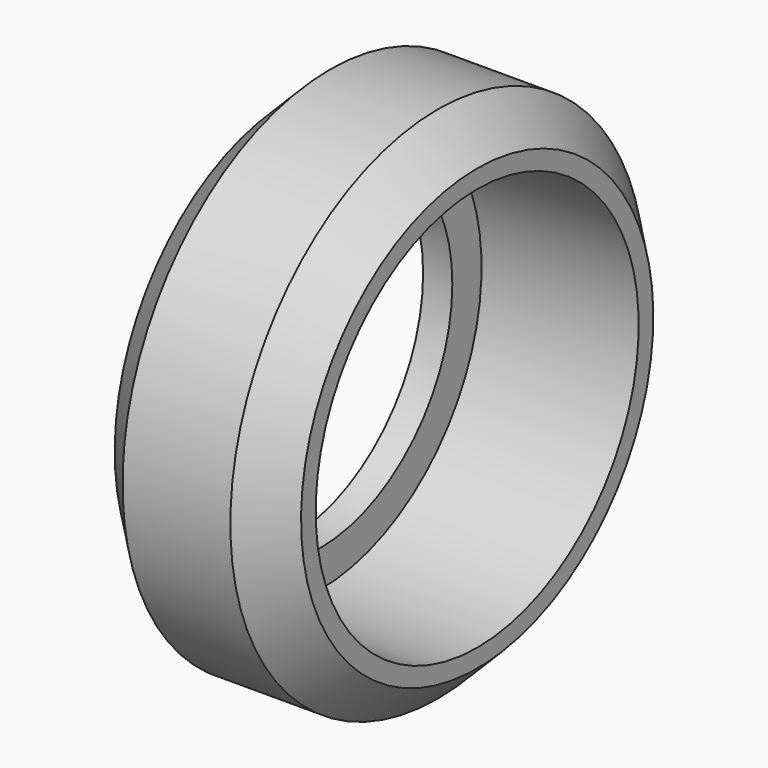
from build123d import *

# Parameters (mm, degrees)
F0_W = 1.6
F0_H = 2


with BuildPart() as f1:
    # F0 (on Front) → F1 (revolve)
    with BuildSketch(Plane.XZ):
        Polygon((-5.1, 12.05), (-5.1, 11.05), (-3.5, 11.05), (5.1, 11.05), (5.1, 12.05), (2.95, 14.2), (-2.95, 14.2), align=None)
        with Locations((-4.3, 10.05)):
            Rectangle(F0_W, F0_H)
    revolve(axis=Axis((3.7481290151, 0, 0), (1, 0, 0)))


solid = f1.part
